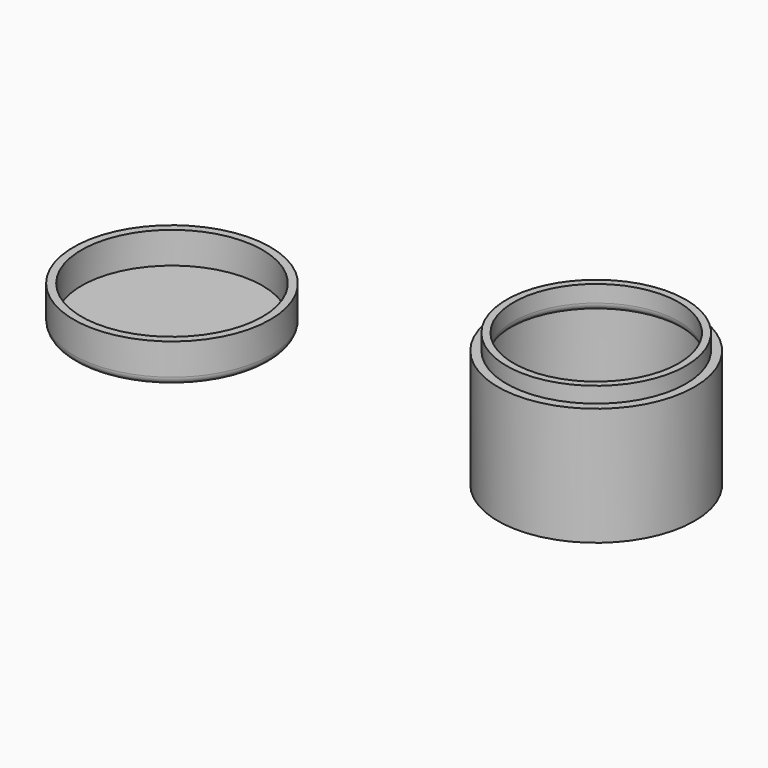
from build123d import *

# Parameters (mm, degrees)
F0_R      = 12.5
F1_DEPTH  = 15
F2_T      = -1.5
F3_R      = 11.4
F3_R_2    = 11
F4_DEPTH  = 2
F5_R      = 12.5
F6_DEPTH  = 5
F7_T      = -1
F8_R      = 1
F10_R     = 11
F10_R_2   = 10.5
F11_DEPTH = 3


# Not quite as in the source:
# - a fillet or chamfer that OpenCascade refuses, or shapes differently, is made with other operations: its cross-section is extruded or revolved along the edge and cut away or added


with BuildPart() as f1:
    # F0 (on Top) → F1 (new body)
    with BuildSketch(Plane.XY):
        Circle(F0_R)
    extrude(amount=F1_DEPTH)

    # F2
    f2_openings = [f1.faces().sort_by_distance(p)[0] for p in [
        (0, 0, 15),
    ]]
    offset(amount=F2_T, openings=f2_openings)

    # F3 (on face) → F4 (join)
    with BuildSketch(Plane.XY.offset(15)):
        Circle(F3_R)
        Circle(F3_R_2, mode=Mode.SUBTRACT)
    extrude(amount=F4_DEPTH)

    # F10 (on face) → F11 (join)
    with BuildSketch(Plane.XY.offset(17)):
        Circle(F10_R)
        Circle(F10_R_2, mode=Mode.SUBTRACT)
    extrude(amount=-F11_DEPTH)

    # F12: fillet of radius 1 on 1 edges, made by hand

    # F12_s1 → F12_t2 (revolve, cut)
    with BuildSketch(Plane.XZ):
        with BuildLine():
            ThreePointArc((10.5, 14.8660254038), (10.6339745962, 14.3660254038), (11, 14))
            Line((11, 14), (10.5, 14))
            Line((10.5, 14), (10.5, 14.8660254038))
        make_face()
    revolve(axis=Axis((0, 0, 14), (0, 0, 1)), mode=Mode.SUBTRACT)


with BuildPart() as f6:
    # F5 (on Top) → F6 (new body)
    with BuildSketch(Plane.XY):
        with Locations((-53.9208427072, 0)):
            Circle(F5_R)
    extrude(amount=F6_DEPTH)

    # F7
    f7_openings = [f6.faces().sort_by_distance(p)[0] for p in [
        (-53.920843, 0, 5),
    ]]
    offset(amount=F7_T, openings=f7_openings)

    # F8
    f8_edges = [f6.edges().sort_by_distance(p)[0] for p in [
        (-66.420843, 0, 0),
    ]]
    fillet(f8_edges, radius=F8_R)


solid = Compound([f1.part, f6.part])
